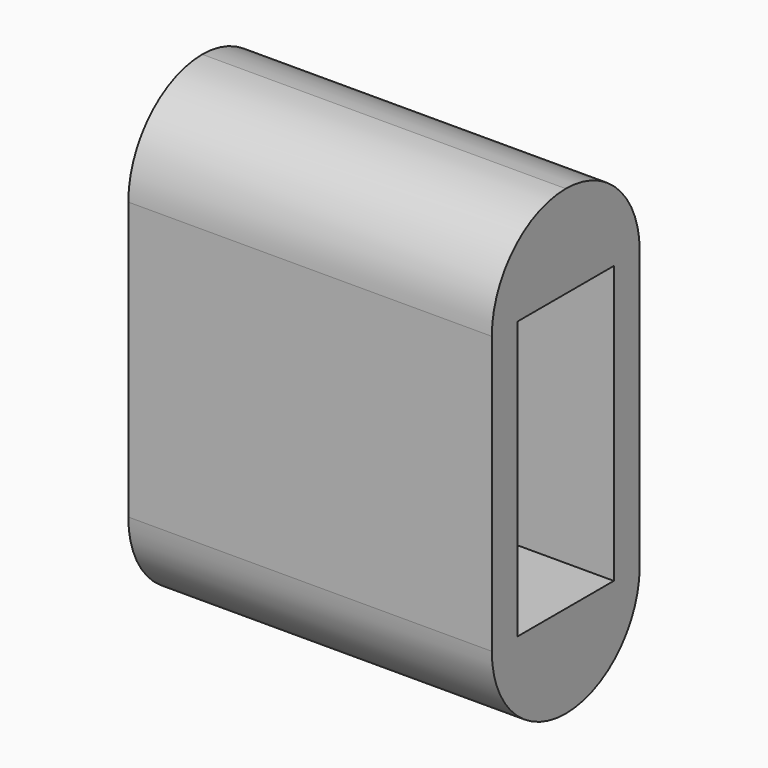
from build123d import *

# Parameters (mm, degrees)
F0_W     = 10.16
F0_H     = 25.4
F0_W_2   = 6.604
F0_H_2   = 15.24
F1_DEPTH = 19.97964
F2_R     = 5.07999


# Not quite as in the source:
# - a fillet or chamfer is up to 0.001 mm smaller than in the source, because OpenCascade refuses the exact size


with BuildPart() as f1:
    # F0 (on Right) → F1 (new body)
    with BuildSketch(Plane.YZ):
        with Locations((6.7968953631, 12.7)):
            Rectangle(F0_W, F0_H)
        with Locations((6.7968953631, 12.7)):
            Rectangle(F0_W_2, F0_H_2, mode=Mode.SUBTRACT)
    extrude(amount=F1_DEPTH)

    # F2 (radius 5.08 in the source; OpenCascade refuses exactly that, so slightly less here)
    f2_edges = [f1.edges().sort_by_distance(p)[0] for p in [
        (9.98982, 1.716895, 25.4),
        (9.98982, 11.876895, 25.4),
        (9.98982, 1.716895, 0),
        (9.98982, 11.876895, 0),
    ]]
    fillet(f2_edges, radius=F2_R)


solid = f1.part
